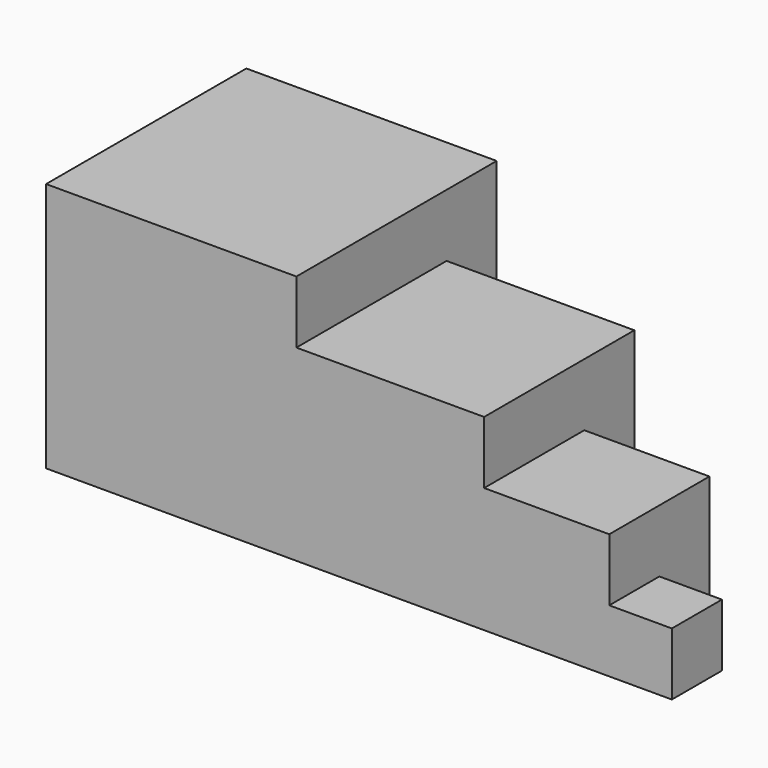
from build123d import *

# Parameters (mm, degrees)
F1_DEPTH    = 4
F2_T4_DEPTH = 24
F3_T4_DEPTH = 19
F4_T4_DEPTH = 14
F5_R        = 0.99999
F7_DEPTH    = 25


# Not quite as in the source:
# - a fillet or chamfer that OpenCascade refuses, or shapes differently, is made with other operations: its cross-section is extruded or revolved along the edge and cut away or added
# - a fillet or chamfer is up to 0.001 mm smaller than in the source, because OpenCascade refuses the exact size


with BuildPart() as f1:
    # F0 (on Top) → F1 (new body)
    with BuildSketch(Plane.XY):
        Polygon((4, 0), (5, 0), (5, 1), (4, 1), (4, 2), (2, 2), (2, 3), (-1, 3), (-1, 4), (-5, 4), (-5, 0), align=None)
        Polygon((-14, 0), (-5, 0), (-5, 4), (-9, 4), (-9, 3), (-12, 3), (-12, 2), (-14, 2), (-14, 1), (-15, 1), (-15, 0), align=None)
    extrude(amount=F1_DEPTH)

    # F2: fillet of radius 4 on 1 edges, made by hand


with BuildPart() as f2_tool2:
    # F2_s3 → F2_t4 (new body)
    with BuildSketch(Plane.XY.offset(-10)):
        with BuildLine():
            ThreePointArc((-5, 4), (-7.8284271247, 2.8284271247), (-9, 0))
            Line((-9, 0), (-9, 4))
            Line((-9, 4), (-5, 4))
        make_face()
    extrude(amount=F2_T4_DEPTH)

    split(bisect_by=Plane.XZ.offset(-3), keep=Keep.BOTTOM)


with BuildPart() as f1_1:
    add(f1.part)

    # F2_t1: cut F2_tool2
    add(f2_tool2.part, mode=Mode.SUBTRACT)

    # F3: fillet of radius 3 on 1 edges, made by hand


with BuildPart() as f3_tool2:
    # F3_s3 → F3_t4 (new body)
    with BuildSketch(Plane.XY.offset(-7.5)):
        with BuildLine():
            ThreePointArc((-12, 0), (-11.1213203436, 2.1213203436), (-9, 3))
            Line((-9, 3), (-12, 3))
            Line((-12, 3), (-12, 0))
        make_face()
    extrude(amount=F3_T4_DEPTH)

    split(bisect_by=Plane.XZ.offset(-2), keep=Keep.BOTTOM)


with BuildPart() as f1_2:
    add(f1_1.part)

    # F3_t1: cut F3_tool2
    add(f3_tool2.part, mode=Mode.SUBTRACT)

    # F4: fillet of radius 2 on 1 edges, made by hand


with BuildPart() as f4_tool2:
    # F4_s3 → F4_t4 (new body)
    with BuildSketch(Plane.XY.offset(-5)):
        with BuildLine():
            ThreePointArc((-14, 0), (-13.4142135624, 1.4142135624), (-12, 2))
            Line((-12, 2), (-14, 2))
            Line((-14, 2), (-14, 0))
        make_face()
    extrude(amount=F4_T4_DEPTH)

    split(bisect_by=Plane.XZ.offset(-1), keep=Keep.BOTTOM)


with BuildPart() as f1_3:
    add(f1_2.part)

    # F4_t1: cut F4_tool2
    add(f4_tool2.part, mode=Mode.SUBTRACT)

    # F5 (radius 1 in the source; OpenCascade refuses exactly that, so slightly less here)
    f5_edges = [f1_3.edges().sort_by_distance(p)[0] for p in [
        (-15, 1, 2),
    ]]
    fillet(f5_edges, radius=F5_R)

    # F6 (on face) → F7 (intersect)
    with BuildSketch(Plane.XZ):
        Polygon((-5, 0), (5, 0), (5, 1), (4, 1), (4, 2), (2, 2), (2, 3), (-1, 3), (-1, 4), (-5, 4), align=None)
    extrude(amount=-F7_DEPTH, mode=Mode.INTERSECT)


solid = f1_3.part
